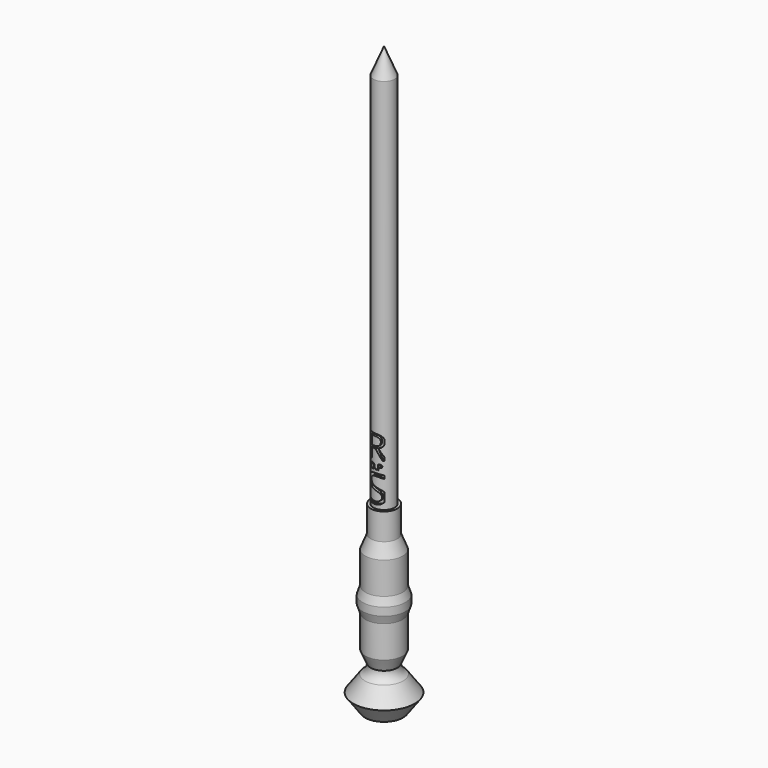
from build123d import *

# Parameters (mm, degrees)
F3_START       = 3
F2_TEXT_SIZE   = 12.0131393712
F2_TEXT_SIZE_2 = 14.1397404032
F2_TEXT_SIZE_3 = 2.7727180471
F3_DEPTH       = 7


# Not quite as in the source:
# - a feature names something its author has since deleted; it is built from what else it names
# - Text() gives the source's letters only with a copy of the font that has no kerning and outlines rounded to 1/6400 em; it was checked with that copy


with BuildPart() as f1:
    # F0 (on Front) → F1 (revolve)
    with BuildSketch(Plane.XZ):
        with BuildLine():
            ThreePointArc((7.1329238722, -111.5481509862), (5.5726925179, -110.0231930885), (5, -107.9179990953))
            Line((5, -107.9179990953), (7, -103.3354234003))
            Line((7, -103.3354234003), (7, -91.3354234003))
            Line((7, -91.3354234003), (8, -88.3354234003))
            Line((8, -88.3354234003), (8, -85.3354234003))
            Line((8, -85.3354234003), (7, -82.3354234003))
            Line((7, -82.3354234003), (7, -70.3354234003))
            Line((7, -70.3354234003), (5, -65.3354234003))
            Line((5, -65.3354234003), (5, -55.3354234003))
            Line((5, -55.3354234003), (4, -55.3354234003))
            Line((4, -55.3354234003), (4, 86.134221556))
            Line((4, 86.134221556), (0, 95.7346098689))
            Line((0, 95.7346098689), (0, 86.134221556))
            Line((0, 86.134221556), (0, -113.865778444))
            Line((0, -113.865778444), (7.1329238722, -111.5481509862))
        make_face()
        Polygon((11.5413132644, -117.615778444), (7.1329238722, -111.5481509862), (0, -113.865778444), (0, -121.365778444), (7.1329238722, -123.6834059018), align=None)
    revolve(axis=Axis((0, 0, -13.865778444), (0, 0, -1)))

    # F2 (on Front) → F3 (cut)
    with BuildSketch(Plane.XZ.offset(F3_START)):
        with Locations((-3.8853062714, -39.1109612773)):
            Text('R', F2_TEXT_SIZE, font='Open Sans', text_align=(TextAlign.LEFT, TextAlign.BOTTOM))
        with Locations((-3.8853062714, -53.7974092114)):
            Text('S', F2_TEXT_SIZE_2, font='Open Sans', text_align=(TextAlign.LEFT, TextAlign.BOTTOM))
        with Locations((-2.3220073126, -42.4372926354)):
            Text('O.P', F2_TEXT_SIZE_3, font='Open Sans', text_align=(TextAlign.LEFT, TextAlign.BOTTOM))
    extrude(amount=F3_DEPTH, mode=Mode.SUBTRACT)


solid = f1.part
